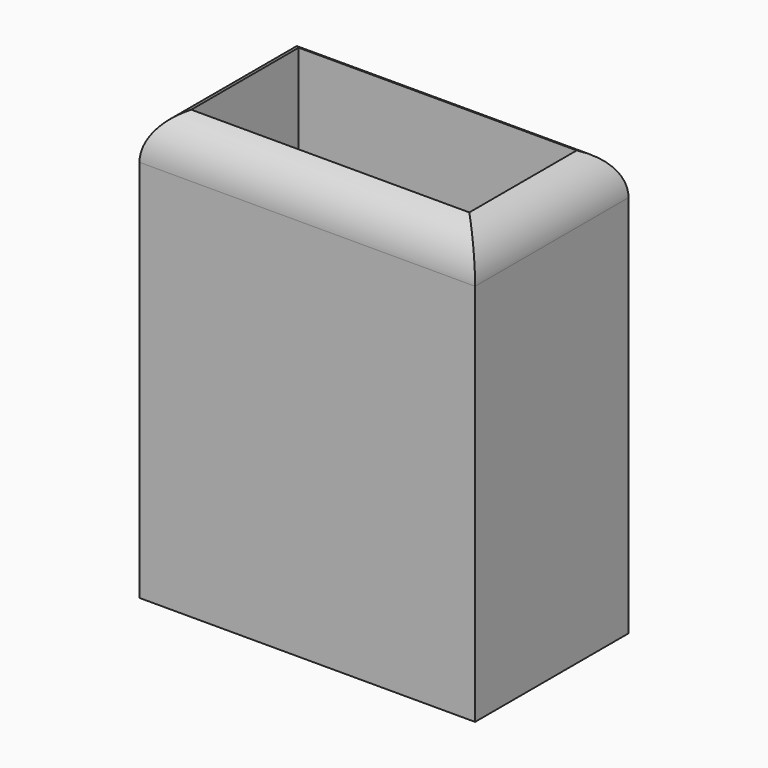
from build123d import *

# Parameters (mm, degrees)
F0_W        = 35
F0_H        = 20
F1_DEPTH    = 45
F2_W        = 29
F2_H        = 14
F3_DEPTH    = 40
F4_T1_DEPTH = 45
F4_T3_DEPTH = 60


# Not quite as in the source:
# - a fillet or chamfer that OpenCascade refuses, or shapes differently, is made with other operations: its cross-section is extruded or revolved along the edge and cut away or added
# - a feature names something its author has since deleted; it is built from what else it names


with BuildPart() as f1:
    # F0 (on Top) → F1 (new body)
    with BuildSketch(Plane.XY):
        Rectangle(F0_W, F0_H)
    extrude(amount=F1_DEPTH)

    # F2 (on face) → F3 (cut)
    with BuildSketch(Plane.XY.offset(45)):
        Rectangle(F2_W, F2_H)
    extrude(amount=-F3_DEPTH, mode=Mode.SUBTRACT)

    # F4: fillet of radius 5 on 4 edges, made by hand

    # F4_s2 → F4_t1 (cut)
    with BuildSketch(Plane.XZ.offset(-22.5)):
        with BuildLine():
            ThreePointArc((17.5, 40), (16.0355339059, 43.5355339059), (12.5, 45))
            Line((12.5, 45), (17.5, 45))
            Line((17.5, 45), (17.5, 40))
        make_face()
        with BuildLine():
            ThreePointArc((-17.5, 40), (-16.0355339059, 43.5355339059), (-12.5, 45))
            Line((-12.5, 45), (-17.5, 45))
            Line((-17.5, 45), (-17.5, 40))
        make_face()
    extrude(amount=F4_T1_DEPTH, mode=Mode.SUBTRACT)

    # F4_s4 → F4_t3 (cut)
    with BuildSketch(Plane.YZ.offset(-30)):
        with BuildLine():
            ThreePointArc((-5, 45), (-8.5355339059, 43.5355339059), (-10, 40))
            Line((-10, 40), (-10, 45))
            Line((-10, 45), (-5, 45))
        make_face()
        with BuildLine():
            ThreePointArc((10, 40), (8.5355339059, 43.5355339059), (5, 45))
            Line((5, 45), (10, 45))
            Line((10, 45), (10, 40))
        make_face()
    extrude(amount=F4_T3_DEPTH, mode=Mode.SUBTRACT)


solid = f1.part
